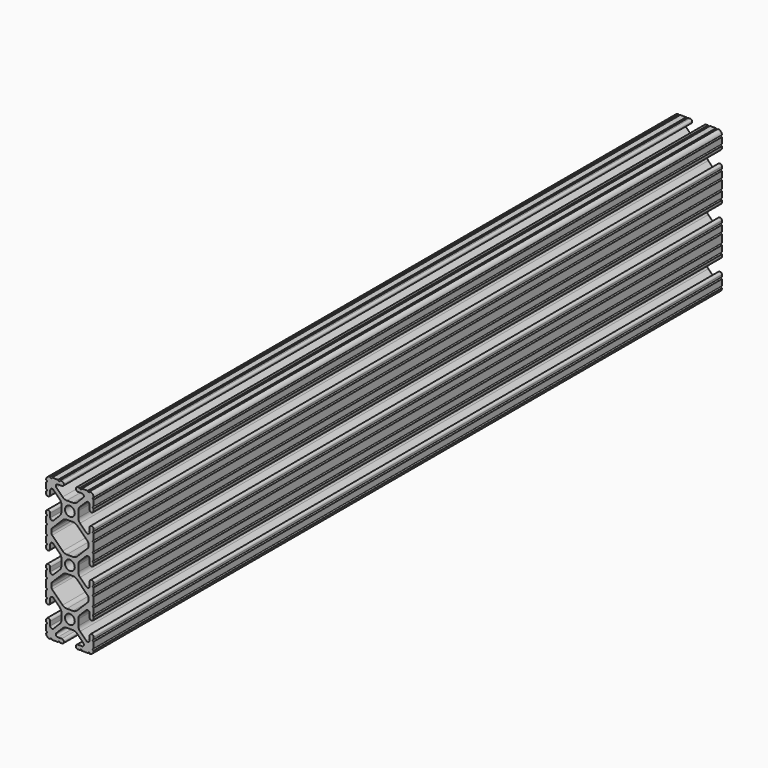
from build123d import *

# Parameters (mm, degrees)
F1_DEPTH = 419


# Not quite as in the source:
# - ends of sketch curves that miss each other by under 0.0002 mm in the source are joined


with BuildPart() as f1:
    # F0 (on Front) → F1 (new body)
    with BuildSketch(Plane.XZ):
        with BuildLine():
            ThreePointArc((-9.5504, 38.1), (-10.0584, 37.592), (-10.5664, 38.1))
            ThreePointArc((-10.5664, 38.1), (-12.0826749161, 37.4826749161), (-12.699997541, 35.9664000298))
            ThreePointArc((-12.699997541, 35.9664000298), (-12.192, 35.4584), (-12.7, 34.9504))
            Line((-12.7, 34.9504), (-12.7, 31.7246))
            ThreePointArc((-12.7, 31.7246), (-12.192, 31.2166), (-12.7, 30.7086))
            Line((-12.7, 30.7086), (-12.7, 29.7023028))
            ThreePointArc((-12.7, 29.7023028), (-11.5951, 28.5974028), (-10.4902, 29.7023028))
            Line((-10.4902, 29.7023028), (-10.4902, 31.8747902))
            ThreePointArc((-10.4902, 31.8747902), (-9.8630063673, 32.813451805), (-8.7557795103, 32.5932106897))
            Line((-8.7557795103, 32.5932106897), (-5.4384448, 29.2758622))
            ThreePointArc((-5.4384448, 29.2758622), (-4.7501824843, 28.2458268978), (-4.5085, 27.030807))
            Line((-4.5085, 27.030807), (-4.5085, 23.769193))
            ThreePointArc((-4.5085, 23.769193), (-4.7501824843, 22.5541731022), (-5.4384359697, 21.5241289697))
            Line((-5.4384359697, 21.5241289697), (-8.7557864, 18.2067962))
            ThreePointArc((-8.7557864, 18.2067962), (-9.8630063673, 17.986548195), (-10.4902, 18.9252098))
            Line((-10.4902, 18.9252098), (-10.4902, 21.0976972))
            ThreePointArc((-10.4902, 21.0976972), (-11.5951, 22.2025972), (-12.7, 21.0976972))
            Line((-12.7, 21.0976972), (-12.7, 20.0914))
            ThreePointArc((-12.7, 20.0914), (-12.192, 19.5834), (-12.7, 19.0754))
            Line((-12.7, 19.0754), (-12.7, 15.8496))
            ThreePointArc((-12.7, 15.8496), (-12.192, 15.3416), (-12.7, 14.8336))
            Line((-12.7, 14.8336), (-12.7, 10.5664))
            ThreePointArc((-12.7, 10.5664), (-12.192, 10.0584), (-12.7, 9.5504))
            Line((-12.7, 9.5504), (-12.7, 6.3246))
            ThreePointArc((-12.7, 6.3246), (-12.192, 5.8166), (-12.7, 5.3086))
            Line((-12.7, 5.3086), (-12.7, 4.3023028))
            ThreePointArc((-12.7, 4.3023028), (-11.5951, 3.1974028), (-10.4902, 4.3023028))
            Line((-10.4902, 4.3023028), (-10.4902, 6.4747902))
            ThreePointArc((-10.4902, 6.4747902), (-9.8630063673, 7.413451805), (-8.7557795103, 7.1932106897))
            Line((-8.7557795103, 7.1932106897), (-5.4384448, 3.8758622))
            ThreePointArc((-5.4384448, 3.8758622), (-4.7501824843, 2.8458268978), (-4.5085, 1.630807))
            Line((-4.5085, 1.630807), (-4.5085, -1.630807))
            ThreePointArc((-4.5085, -1.630807), (-4.7501824843, -2.8458268978), (-5.4384359697, -3.8758710303))
            Line((-5.4384359697, -3.8758710303), (-8.7557864, -7.1932038))
            ThreePointArc((-8.7557864, -7.1932038), (-9.8630063673, -7.413451805), (-10.4902, -6.4747902))
            Line((-10.4902, -6.4747902), (-10.4902, -4.3023028))
            ThreePointArc((-10.4902, -4.3023028), (-11.5951, -3.1974028), (-12.7, -4.3023028))
            Line((-12.7, -4.3023028), (-12.7, -5.3086))
            ThreePointArc((-12.7, -5.3086), (-12.192, -5.8166), (-12.7, -6.3246))
            Line((-12.7, -6.3246), (-12.7, -9.5504))
            ThreePointArc((-12.7, -9.5504), (-12.192, -10.0584), (-12.7, -10.5664))
            Line((-12.7, -10.5664), (-12.7, -14.8336))
            ThreePointArc((-12.7, -14.8336), (-12.192, -15.3416), (-12.7, -15.8496))
            Line((-12.7, -15.8496), (-12.7, -19.0754))
            ThreePointArc((-12.7, -19.0754), (-12.192, -19.5834), (-12.7, -20.0914))
            Line((-12.7, -20.0914), (-12.7, -21.0976972))
            ThreePointArc((-12.7, -21.0976972), (-11.5951, -22.2025972), (-10.4902, -21.0976972))
            Line((-10.4902, -21.0976972), (-10.4902, -18.9252098))
            ThreePointArc((-10.4902, -18.9252098), (-9.8630063673, -17.986548195), (-8.7557795103, -18.2067893103))
            Line((-8.7557795103, -18.2067893103), (-5.4384448, -21.5241378))
            ThreePointArc((-5.4384448, -21.5241378), (-4.7501824843, -22.5541731022), (-4.5085, -23.769193))
            Line((-4.5085, -23.769193), (-4.5085, -27.030807))
            ThreePointArc((-4.5085, -27.030807), (-4.7501824843, -28.2458268978), (-5.4384359697, -29.2758710303))
            Line((-5.4384359697, -29.2758710303), (-8.7557864, -32.5932038))
            ThreePointArc((-8.7557864, -32.5932038), (-9.8630063673, -32.813451805), (-10.4902, -31.8747902))
            Line((-10.4902, -31.8747902), (-10.4902, -29.7023028))
            ThreePointArc((-10.4902, -29.7023028), (-11.5951, -28.5974028), (-12.7, -29.7023028))
            Line((-12.7, -29.7023028), (-12.7, -30.7086))
            ThreePointArc((-12.7, -30.7086), (-12.192, -31.2166), (-12.7, -31.7246))
            Line((-12.7, -31.7246), (-12.7, -34.9504))
            ThreePointArc((-12.7, -34.9504), (-12.192, -35.4584), (-12.7, -35.9664))
            ThreePointArc((-12.7, -35.9664), (-12.0826749161, -37.4826749161), (-10.5664000298, -38.099997541))
            ThreePointArc((-10.5664000298, -38.099997541), (-10.0584, -37.592), (-9.5504, -38.1))
            Line((-9.5504, -38.1), (-6.3246, -38.1))
            ThreePointArc((-6.3246, -38.1), (-5.8166, -37.592), (-5.3086, -38.1))
            Line((-5.3086, -38.1), (-4.3023028, -38.1))
            ThreePointArc((-4.3023028, -38.1), (-3.1974028, -36.9951), (-4.3023028, -35.8902))
            Line((-4.3023028, -35.8902), (-6.4747902, -35.8902))
            ThreePointArc((-6.4747902, -35.8902), (-7.413451805, -35.2630063673), (-7.1932106897, -34.1557795103))
            Line((-7.1932106897, -34.1557795103), (-3.8758622, -30.8384448))
            ThreePointArc((-3.8758622, -30.8384448), (-2.8458268978, -30.1501824843), (-1.630807, -29.9085))
            Line((-1.630807, -29.9085), (1.630807, -29.9085))
            ThreePointArc((1.630807, -29.9085), (2.8458268978, -30.1501824843), (3.8758710303, -30.8384359697))
            Line((3.8758710303, -30.8384359697), (7.1932038, -34.1557864))
            ThreePointArc((7.1932038, -34.1557864), (7.413451805, -35.2630063673), (6.4747902, -35.8902))
            Line((6.4747902, -35.8902), (4.3023028, -35.8902))
            ThreePointArc((4.3023028, -35.8902), (3.1974028, -36.9951), (4.3023028, -38.1))
            Line((4.3023028, -38.1), (5.3086, -38.1))
            ThreePointArc((5.3086, -38.1), (5.8166, -37.592), (6.3246, -38.1))
            Line((6.3246, -38.1), (9.5504, -38.1))
            ThreePointArc((9.5504, -38.1), (10.0584, -37.592), (10.5664, -38.1))
            ThreePointArc((10.5664, -38.1), (12.0826749161, -37.4826749161), (12.699997541, -35.9664000298))
            ThreePointArc((12.699997541, -35.9664000298), (12.192, -35.4584), (12.7, -34.9504))
            Line((12.7, -34.9504), (12.7, -31.7246))
            ThreePointArc((12.7, -31.7246), (12.192, -31.2166), (12.7, -30.7086))
            Line((12.7, -30.7086), (12.7, -29.7023028))
            ThreePointArc((12.7, -29.7023028), (11.5951, -28.5974028), (10.4902, -29.7023028))
            Line((10.4902, -29.7023028), (10.4902, -31.8747902))
            ThreePointArc((10.4902, -31.8747902), (9.8630063673, -32.813451805), (8.7557795103, -32.5932106897))
            Line((8.7557795103, -32.5932106897), (5.4384448, -29.2758622))
            ThreePointArc((5.4384448, -29.2758622), (4.7501824843, -28.2458268978), (4.5085, -27.030807))
            Line((4.5085, -27.030807), (4.5085, -23.769193))
            ThreePointArc((4.5085, -23.769193), (4.7501824843, -22.5541731022), (5.4384359697, -21.5241289697))
            Line((5.4384359697, -21.5241289697), (8.7557864, -18.2067962))
            ThreePointArc((8.7557864, -18.2067962), (9.8630063673, -17.986548195), (10.4902, -18.9252098))
            Line((10.4902, -18.9252098), (10.4902, -21.0976972))
            ThreePointArc((10.4902, -21.0976972), (11.5951, -22.2025972), (12.7, -21.0976972))
            Line((12.7, -21.0976972), (12.7, -20.0914))
            ThreePointArc((12.7, -20.0914), (12.192, -19.5834), (12.7, -19.0754))
            Line((12.7, -19.0754), (12.7, -15.8496))
            ThreePointArc((12.7, -15.8496), (12.192, -15.3416), (12.7, -14.8336))
            Line((12.7, -14.8336), (12.7, -10.5664))
            ThreePointArc((12.7, -10.5664), (12.192, -10.0584), (12.7, -9.5504))
            Line((12.7, -9.5504), (12.7, -6.3246))
            ThreePointArc((12.7, -6.3246), (12.192, -5.8166), (12.7, -5.3086))
            Line((12.7, -5.3086), (12.7, -4.3023028))
            ThreePointArc((12.7, -4.3023028), (11.5951, -3.1974028), (10.4902, -4.3023028))
            Line((10.4902, -4.3023028), (10.4902, -6.4747902))
            ThreePointArc((10.4902, -6.4747902), (9.8630063673, -7.413451805), (8.7557795103, -7.1932106897))
            Line((8.7557795103, -7.1932106897), (5.4384448, -3.8758622))
            ThreePointArc((5.4384448, -3.8758622), (4.7501824843, -2.8458268978), (4.5085, -1.630807))
            Line((4.5085, -1.630807), (4.5085, 1.630807))
            ThreePointArc((4.5085, 1.630807), (4.7501824843, 2.8458268978), (5.4384359697, 3.8758710303))
            Line((5.4384359697, 3.8758710303), (8.7557864, 7.1932038))
            ThreePointArc((8.7557864, 7.1932038), (9.8630063673, 7.413451805), (10.4902, 6.4747902))
            Line((10.4902, 6.4747902), (10.4902, 4.3023028))
            ThreePointArc((10.4902, 4.3023028), (11.5951, 3.1974028), (12.7, 4.3023028))
            Line((12.7, 4.3023028), (12.7, 5.3086))
            ThreePointArc((12.7, 5.3086), (12.192, 5.8166), (12.7, 6.3246))
            Line((12.7, 6.3246), (12.7, 9.5504))
            ThreePointArc((12.7, 9.5504), (12.192, 10.0584), (12.7, 10.5664))
            Line((12.7, 10.5664), (12.7, 14.8336))
            ThreePointArc((12.7, 14.8336), (12.192, 15.3416), (12.7, 15.8496))
            Line((12.7, 15.8496), (12.7, 19.0754))
            ThreePointArc((12.7, 19.0754), (12.192, 19.5834), (12.7, 20.0914))
            Line((12.7, 20.0914), (12.7, 21.0976972))
            ThreePointArc((12.7, 21.0976972), (11.5951, 22.2025972), (10.4902, 21.0976972))
            Line((10.4902, 21.0976972), (10.4902, 18.9252098))
            ThreePointArc((10.4902, 18.9252098), (9.8630063673, 17.986548195), (8.7557795103, 18.2067893103))
            Line((8.7557795103, 18.2067893103), (5.4384448, 21.5241378))
            ThreePointArc((5.4384448, 21.5241378), (4.7501824843, 22.5541731022), (4.5085, 23.769193))
            Line((4.5085, 23.769193), (4.5085, 27.030807))
            ThreePointArc((4.5085, 27.030807), (4.7501824843, 28.2458268978), (5.4384359697, 29.2758710303))
            Line((5.4384359697, 29.2758710303), (8.7557864, 32.5932038))
            ThreePointArc((8.7557864, 32.5932038), (9.8630063673, 32.813451805), (10.4902, 31.8747902))
            Line((10.4902, 31.8747902), (10.4902, 29.7023028))
            ThreePointArc((10.4902, 29.7023028), (11.5951, 28.5974028), (12.7, 29.7023028))
            Line((12.7, 29.7023028), (12.7, 30.7086))
            ThreePointArc((12.7, 30.7086), (12.192, 31.2166), (12.7, 31.7246))
            Line((12.7, 31.7246), (12.7, 34.9504))
            ThreePointArc((12.7, 34.9504), (12.192, 35.4584), (12.7, 35.9664))
            ThreePointArc((12.7, 35.9664), (12.0826749161, 37.4826749161), (10.5664000298, 38.099997541))
            ThreePointArc((10.5664000298, 38.099997541), (10.0584, 37.592), (9.5504, 38.1))
            Line((9.5504, 38.1), (6.3246, 38.1))
            ThreePointArc((6.3246, 38.1), (5.8166, 37.592), (5.3086, 38.1))
            Line((5.3086, 38.1), (4.3023028, 38.1))
            ThreePointArc((4.3023028, 38.1), (3.1974028, 36.9951), (4.3023028, 35.8902))
            Line((4.3023028, 35.8902), (6.4747902, 35.8902))
            ThreePointArc((6.4747902, 35.8902), (7.413451805, 35.2630063673), (7.1932106897, 34.1557795103))
            Line((7.1932106897, 34.1557795103), (3.8758622, 30.8384448))
            ThreePointArc((3.8758622, 30.8384448), (2.8458268978, 30.1501824843), (1.630807, 29.9085))
            Line((1.630807, 29.9085), (-1.630807, 29.9085))
            ThreePointArc((-1.630807, 29.9085), (-2.8458268978, 30.1501824843), (-3.8758710303, 30.8384359697))
            Line((-3.8758710303, 30.8384359697), (-7.1932038, 34.1557864))
            ThreePointArc((-7.1932038, 34.1557864), (-7.413451805, 35.2630063673), (-6.4747902, 35.8902))
            Line((-6.4747902, 35.8902), (-4.3023028, 35.8902))
            ThreePointArc((-4.3023028, 35.8902), (-3.1974028, 36.9951), (-4.3023028, 38.1))
            Line((-4.3023028, 38.1), (-5.3086, 38.1))
            ThreePointArc((-5.3086, 38.1), (-5.8166, 37.592), (-6.3246, 38.1))
            Line((-6.3246, 38.1), (-9.5504, 38.1))
        make_face()
        with BuildLine():
            ThreePointArc((-2.6035, -25.4), (0, -22.7965), (2.6035, -25.4))
            ThreePointArc((2.6035, -25.4), (0, -28.0035), (-2.6035, -25.4))
        make_face(mode=Mode.SUBTRACT)
        with BuildLine():
            Line((-9.4701614, -11.0327186), (-3.8758622, -5.4384448))
            ThreePointArc((-3.8758622, -5.4384448), (-2.8458268978, -4.7501824843), (-1.630807, -4.5085))
            Line((-1.630807, -4.5085), (1.630807, -4.5085))
            ThreePointArc((1.630807, -4.5085), (2.8458268978, -4.7501824843), (3.8758710303, -5.4384359697))
            Line((3.8758710303, -5.4384359697), (9.4701614, -11.0327186))
            ThreePointArc((9.4701614, -11.0327186), (9.8115254878, -11.5436301307), (9.9314, -12.14628))
            Line((9.9314, -12.14628), (9.9314, -13.25372))
            ThreePointArc((9.9314, -13.25372), (9.8115254878, -13.8563698693), (9.470151759, -14.367271759))
            Line((9.470151759, -14.367271759), (3.8758622, -19.9615552))
            ThreePointArc((3.8758622, -19.9615552), (2.8458268978, -20.6498175157), (1.630807, -20.8915))
            Line((1.630807, -20.8915), (-1.630807, -20.8915))
            ThreePointArc((-1.630807, -20.8915), (-2.8458268978, -20.6498175157), (-3.8758710303, -19.9615640303))
            Line((-3.8758710303, -19.9615640303), (-9.4701614, -14.3672814))
            ThreePointArc((-9.4701614, -14.3672814), (-9.8115254878, -13.8563698693), (-9.9314, -13.25372))
            Line((-9.9314, -13.25372), (-9.9314, -12.14628))
            ThreePointArc((-9.9314, -12.14628), (-9.8115254878, -11.5436301307), (-9.4701614, -11.0327186))
        make_face(mode=Mode.SUBTRACT)
        with BuildLine():
            ThreePointArc((-2.6035, 0), (0, 2.6035), (2.6035, 0))
            ThreePointArc((2.6035, 0), (0, -2.6035), (-2.6035, 0))
        make_face(mode=Mode.SUBTRACT)
        with BuildLine():
            Line((-9.4701614, 14.3672814), (-3.8758622, 19.9615552))
            ThreePointArc((-3.8758622, 19.9615552), (-2.8458268978, 20.6498175157), (-1.630807, 20.8915))
            Line((-1.630807, 20.8915), (1.630807, 20.8915))
            ThreePointArc((1.630807, 20.8915), (2.8458268978, 20.6498175157), (3.8758710303, 19.9615640303))
            Line((3.8758710303, 19.9615640303), (9.4701614, 14.3672814))
            ThreePointArc((9.4701614, 14.3672814), (9.8115254878, 13.8563698693), (9.9314, 13.25372))
            Line((9.9314, 13.25372), (9.9314, 12.14628))
            ThreePointArc((9.9314, 12.14628), (9.8115254878, 11.5436301307), (9.470151759, 11.032728241))
            Line((9.470151759, 11.032728241), (3.8758622, 5.4384448))
            ThreePointArc((3.8758622, 5.4384448), (2.8458268978, 4.7501824843), (1.630807, 4.5085))
            Line((1.630807, 4.5085), (-1.630807, 4.5085))
            ThreePointArc((-1.630807, 4.5085), (-2.8458268978, 4.7501824843), (-3.8758710303, 5.4384359697))
            Line((-3.8758710303, 5.4384359697), (-9.4701614, 11.0327186))
            ThreePointArc((-9.4701614, 11.0327186), (-9.8115254878, 11.5436301307), (-9.9314, 12.14628))
            Line((-9.9314, 12.14628), (-9.9314, 13.25372))
            ThreePointArc((-9.9314, 13.25372), (-9.8115254878, 13.8563698693), (-9.4701614, 14.3672814))
        make_face(mode=Mode.SUBTRACT)
        with BuildLine():
            ThreePointArc((-2.6035, 25.4), (0, 28.0035), (2.6035, 25.4))
            ThreePointArc((2.6035, 25.4), (0, 22.7965), (-2.6035, 25.4))
        make_face(mode=Mode.SUBTRACT)
    extrude(amount=F1_DEPTH)


solid = f1.part
